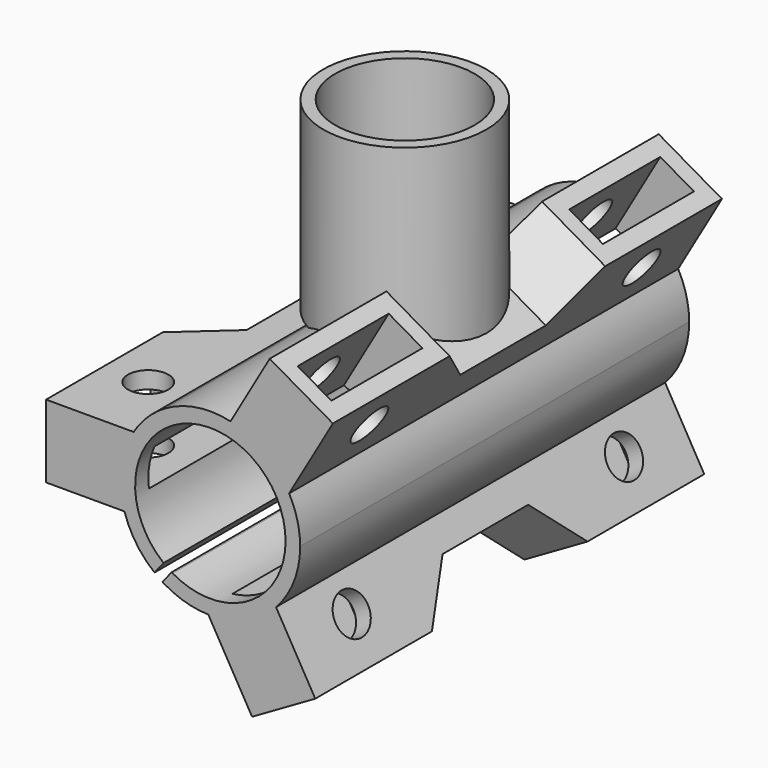
from build123d import *
from build123d import SkipClean  # not in build123d's __all__

# Parameters (mm, degrees)
F0_R      = 4.16
F1_DEPTH  = 15
F3_DEPTH  = 100
F4_W      = 23.4
F4_H      = 8
F5_DEPTH  = 25
F7_COUNT  = 3
F9_START  = 22
F8_R      = 16.7795
F8_R_2    = 13.7795
F9_DEPTH  = 38
F10_R     = 13.7795
F11_DEPTH = 40
F12_R     = 14.33068
F12_R_2   = 13.7795
F13_DEPTH = 40
F15_DEPTH = 100


# Not quite as in the source:
# - a feature names something its author has since deleted; it is built from what else it names


with BuildPart() as f1:
    # F0 (on Top) → F1 (new body)
    with BuildSketch(Plane.XY):
        Polygon((-33.7795, 0), (-15.7795, 0), (-15.7795, 50), (-15.7795, 100), (-33.7795, 100), (-33.7795, 70), (-23.7483102828, 61), (-23.7483102828, 50), (-23.7483102828, 39), (-33.7795, 30), align=None)
        with Locations((-24.7795, 15)):
            Circle(F0_R, mode=Mode.SUBTRACT)
        with Locations((-24.7795, 85)):
            Circle(F0_R, mode=Mode.SUBTRACT)
    extrude(amount=F1_DEPTH)

    # F2 (on face) → F3 (join)
    with BuildSketch(Plane.XZ):
        with BuildLine():
            ThreePointArc((-7.7342375, -7.9925473083), (-15.468475, 5.4035449996), (-7.7342375, 18.7996373074))
            Line((-7.7342375, 18.7996373074), (-9.2342375, 21.3977135187))
            ThreePointArc((-9.2342375, 21.3977135187), (-12.9094713485, 18.6107444881), (-15.7795, 15))
            Line((-15.7795, 15), (-15.7795, 0))
            Line((-15.7795, 0), (-17.6603021, 0))
            ThreePointArc((-17.6603021, 0), (-14.4523144066, -6.0949408624), (-9.2342375, -10.5906235196))
            Line((-9.2342375, -10.5906235196), (-7.7342375, -7.9925473083))
        make_face()
    extrude(amount=-F3_DEPTH)

    # F4 (on face) → F5 (cut)
    with BuildSketch(Plane(origin=(-33.7795, 0, 0), x_dir=(0, -1, 0), z_dir=(-1, 0, 0))):
        with Locations((-84.9, 7.5)):
            Rectangle(F4_W, F4_H)
        with Locations((-15.1, 7.5)):
            Rectangle(F4_W, F4_H)
    extrude(amount=-F5_DEPTH, mode=Mode.SUBTRACT)

    # F7: F1 ×3 about axis
    f7_axis = Axis((0, 0, 5.4035449996), (0, -1, 0))


with BuildPart() as f1_1:
    add(f1.part, clean=False)
    with SkipClean():  # cleaning this boolean's faces spoils the solid; the shape is the same uncleaned
        for i in range(1, F7_COUNT):
            add(f1.part.rotate(f7_axis, i * 360 / F7_COUNT), clean=False)

    # F8 (on Top) → F9 (join)
    with BuildSketch(Plane.XY.offset(F9_START)):
        with Locations((0, 50)):
            Circle(F8_R)
        with Locations((0, 50)):
            Circle(F8_R_2, mode=Mode.SUBTRACT)
    with SkipClean():  # cleaning this boolean's faces spoils the solid; the shape is the same uncleaned
        extrude(amount=F9_DEPTH)

    # F10 (on face) → F11 (cut)
    with BuildSketch(Plane.XY.offset(60)):
        with Locations((0, 50)):
            Circle(F10_R)
    with SkipClean():  # cleaning this boolean's faces spoils the solid; the shape is the same uncleaned
        extrude(amount=-F11_DEPTH, mode=Mode.SUBTRACT)

    # F12 (on face) → F13 (cut)
    with BuildSketch(Plane.XY.offset(60)):
        with Locations((0, 50)):
            Circle(F12_R)
        with Locations((0, 50)):
            Circle(F12_R_2, mode=Mode.SUBTRACT)
    with SkipClean():  # cleaning this boolean's faces spoils the solid; the shape is the same uncleaned
        extrude(amount=-F13_DEPTH, mode=Mode.SUBTRACT)

    # F14 (on Front) → F15 (cut)
    with BuildSketch(Plane.XZ):
        Polygon((-4.9232800736, -4.035219008), (-6.6853797605, -3.0374381485), (-13.2133684748, -11.2353765363), (-11.6488082544, -12.4812301861), align=None)
    extrude(amount=-F15_DEPTH, mode=Mode.SUBTRACT)


solid = f1_1.part
